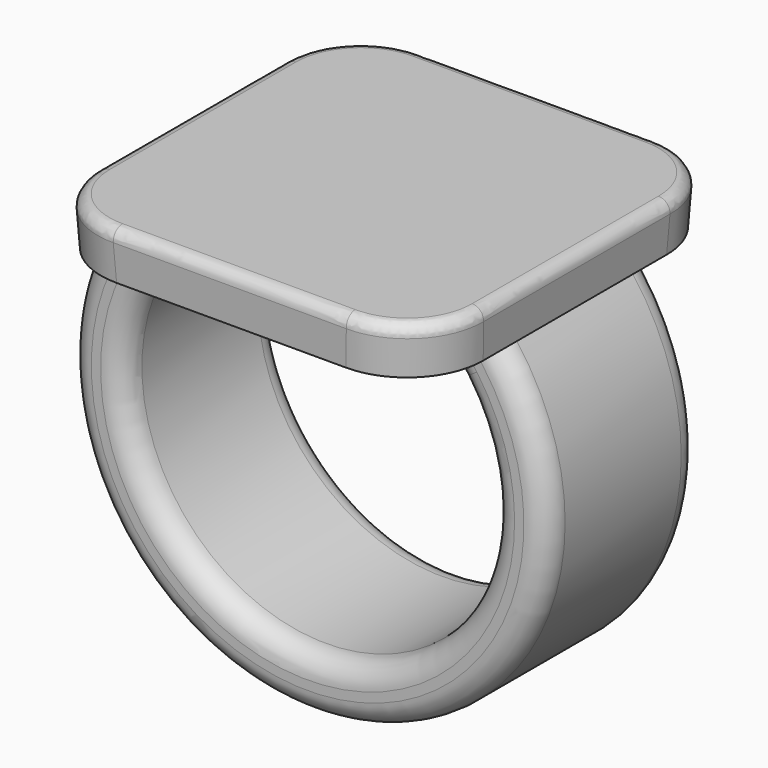
from build123d import *

# Parameters (mm, degrees)
F0_W          = 25.4
F0_H          = 25.4
F1_DEPTH      = 3.175
F1_TAPER      = -3
F3_W          = 5.08
F3_H          = 12.7
F6_DEPTH      = 6.35
F6_DEPTH_BACK = 6.35
F7_R          = 5.08
F8_R          = 1.524
F9_R          = 0.762


with BuildPart() as f1:
    # F0 (on Top) → F1 (new body)
    with BuildSketch(Plane.XY):
        Rectangle(F0_W, F0_H)
    extrude(amount=F1_DEPTH, taper=F1_TAPER)

    # F4: sweep along a path in F2
    with BuildLine(Plane.XZ) as f4_path:
        ThreePointArc((-10.16, 0), (0, -23.5582897328), (10.16, 0))
    # F3 (on face) → F4 (sweep)
    with BuildSketch(Plane(origin=(0, 0, 0), x_dir=(1, 0, 0), z_dir=(0, 0, -1))):
        with Locations((-10.16, 0)):
            Rectangle(F3_W, F3_H)
    sweep(path=f4_path.line)

    # F5 (on Front) → F6 (join, two sides)
    with BuildSketch(Plane.XZ) as f6_sk:
        with BuildLine():
            Line((10.0130578512, -2.535746045), (10.16, 0))
            Line((10.16, 0), (7.62, 0))
            ThreePointArc((7.62, 0), (8.9072265211, -1.1822790439), (10.0130578512, -2.535746045))
        make_face()
    extrude(amount=F6_DEPTH)
    extrude(f6_sk.sketch, amount=-F6_DEPTH_BACK)

    # F7
    f7_edges = [f1.edges().sort_by_distance(p)[0] for p in [
        (12.783197, -12.783197, 1.5875),
        (-12.783197, -12.783197, 1.5875),
        (12.783197, 12.783197, 1.5875),
        (-12.783197, 12.783197, 1.5875),
    ]]
    fillet(f7_edges, radius=F7_R)

    # F8
    f8_edges = [f1.edges().sort_by_distance(p)[0] for p in [
        (-1.743325, 6.35, -21.711017),
        (-1.743325, -6.35, -21.711017),
        (8.907227, -6.35, -1.182279),
        (0, 6.35, -25.501344),
        (0, -6.35, -25.501344),
        (8.907227, 6.35, -1.182279),
    ]]
    fillet(f8_edges, radius=F8_R)

    # F9
    f9_edges = [f1.edges().sort_by_distance(p)[0] for p in [
        (12.866395, 0, 3.175),
        (11.381378, -11.381378, 3.175),
        (11.381378, 11.381378, 3.175),
        (0, -12.866395, 3.175),
        (0, 12.866395, 3.175),
        (-11.381378, -11.381378, 3.175),
        (-11.381378, 11.381378, 3.175),
        (-12.866395, 0, 3.175),
    ]]
    fillet(f9_edges, radius=F9_R)


solid = f1.part
